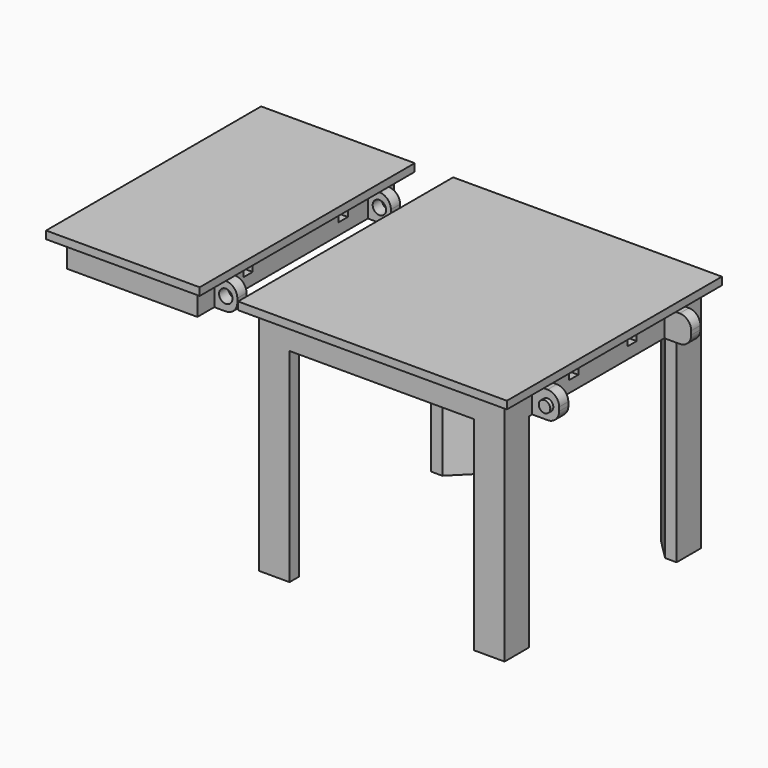
from build123d import *

# Parameters (mm, degrees)
F0_W      = 3
F0_H      = 50
F0_W_2    = 48
F0_H_2    = 3
F0_H_3    = 40
F1_DEPTH  = 2
F2_DEPTH  = 60
F0_W_3    = 4
F3_DEPTH  = 7
F4_R      = 1.25
F4_R_2    = 1.5
F5_DEPTH  = 1
F6_R      = 1.25
F6_R_2    = 1.5
F7_DEPTH  = 1
F8_W      = 28
F8_H      = 58
F8_W_2    = 3
F8_H_2    = 47
F8_H_3    = 3
F9_DEPTH  = 2
F10_DEPTH = 7
F11_DEPTH = 7
F12_R     = 1.75
F13_DEPTH = 61.501
F14_W     = 3
F14_H     = 4
F15_DEPTH = 52.7474034429
F16_R     = 3
F16_2_R   = 3
F17_R     = 2.99999
F17_2_R   = 2.99999
F18_W     = 3
F18_H     = 4
F19_DEPTH = 33.2525965571


# Not quite as in the source:
# - a fillet or chamfer is up to 0.001 mm smaller than in the source, because OpenCascade refuses the exact size


with BuildPart() as f1:
    # F0 (on Top) → F1 (new body)
    with BuildSketch(Plane.XY):
        Polygon((11, -6), (6, -11), (6, -59), (11, -64), (59, -64), (64, -59), (64, -11), (59, -6), align=None)
        with Locations((35.2474034429, -35)):
            Rectangle(F0_W, F0_H, mode=Mode.SUBTRACT)
        Polygon((67, -15), (67, -12), (67, -11), (64, -11), (64, -59), (67, -59), (67, -58), (67, -55), align=None)
        Polygon((70, 0), (0, 0), (0, -12), (3, -12), (3, -11), (3, -3), (11, -3), (59, -3), (67, -3), (67, -11), (67, -12), (70, -12), align=None)
        Polygon((3, -11), (3, -12), (3, -15), (3, -55), (3, -58), (3, -59), (6, -59), (6, -11), align=None)
        with Locations((35, -65.5)):
            Rectangle(F0_W_2, F0_H_2)
        Polygon((67, -59), (64, -59), (59, -64), (59, -67), (67, -67), align=None)
        Polygon((11, -64), (6, -59), (3, -59), (3, -67), (11, -67), align=None)
        Polygon((64, -11), (67, -11), (67, -3), (59, -3), (59, -6), align=None)
        with Locations((35, -4.5)):
            Rectangle(F0_W_2, F0_H_2)
        Polygon((3, -3), (3, -11), (6, -11), (11, -6), (11, -3), align=None)
        with Locations((68.5, -35)):
            Rectangle(F0_W, F0_H_3)
        with Locations((68.5, -13.5)):
            Rectangle(F0_W, F0_H_2)
        with Locations((68.5, -56.5)):
            Rectangle(F0_W, F0_H_2)
        Polygon((3, -58), (0, -58), (0, -70), (70, -70), (70, -58), (67, -58), (67, -59), (67, -67), (59, -67), (11, -67), (3, -67), (3, -59), align=None)
        with Locations((1.5, -35)):
            Rectangle(F0_W, F0_H_3)
        with Locations((1.5, -56.5)):
            Rectangle(F0_W, F0_H_2)
        with Locations((1.5, -13.5)):
            Rectangle(F0_W, F0_H_2)
        with Locations((35.2474034429, -35)):
            Rectangle(F0_W, F0_H)
    extrude(amount=F1_DEPTH)

    # F0 (on Top) → F2 (join)
    with BuildSketch(Plane.XY):
        Polygon((67, -59), (64, -59), (59, -64), (59, -67), (67, -67), align=None)
        Polygon((64, -11), (67, -11), (67, -3), (59, -3), (59, -6), align=None)
        Polygon((3, -3), (3, -11), (6, -11), (11, -6), (11, -3), align=None)
        Polygon((11, -64), (6, -59), (3, -59), (3, -67), (11, -67), align=None)
    extrude(amount=-F2_DEPTH)

    # F0 (on Top) → F3 (join)
    with BuildSketch(Plane.XY):
        Polygon((3, -11), (3, -12), (3, -15), (3, -55), (3, -58), (3, -59), (6, -59), (6, -11), align=None)
        with Locations((-2, -56.5)):
            Rectangle(F0_W_3, F0_H_2)
        with Locations((1.5, -56.5)):
            Rectangle(F0_W, F0_H_2)
        with Locations((1.5, -13.5)):
            Rectangle(F0_W, F0_H_2)
        with Locations((-2, -13.5)):
            Rectangle(F0_W_3, F0_H_2)
        with Locations((35, -65.5)):
            Rectangle(F0_W_2, F0_H_2)
        Polygon((67, -15), (67, -12), (67, -11), (64, -11), (64, -59), (67, -59), (67, -58), (67, -55), align=None)
        with Locations((68.5, -56.5)):
            Rectangle(F0_W, F0_H_2)
        with Locations((72, -56.5)):
            Rectangle(F0_W_3, F0_H_2)
        with Locations((72, -13.5)):
            Rectangle(F0_W_3, F0_H_2)
        with Locations((68.5, -13.5)):
            Rectangle(F0_W, F0_H_2)
        with Locations((35, -4.5)):
            Rectangle(F0_W_2, F0_H_2)
        with Locations((35.2474034429, -35)):
            Rectangle(F0_W, F0_H)
    extrude(amount=-F3_DEPTH)

    # F4 (on face) → F5 (join)
    with BuildSketch(Plane(origin=(0, -12, 0), x_dir=(-1, 0, 0), z_dir=(0, 1, 0))):
        with Locations((1, -3.5)):
            Circle(F4_R)
        with Locations((-71, -3.5)):
            Circle(F4_R_2)
    extrude(amount=F5_DEPTH)

    # F6 (on face) → F7 (join)
    with BuildSketch(Plane.XZ.offset(58)):
        with Locations((0, -3.5)):
            Circle(F6_R)
        with Locations((71, -3.5)):
            Circle(F6_R_2)
    extrude(amount=F7_DEPTH)


with BuildPart() as f9:
    # F8 (on Top) → F9 (new body)
    with BuildSketch(Plane.XY):
        Polygon((-13, -11.5), (-13, -8.5), (-13, -3), (-47, -3), (-47, -67), (-13, -67), (-13, -61.5), (-13, -58.5), align=None)
        with Locations((-30, -35)):
            Rectangle(F8_W, F8_H, mode=Mode.SUBTRACT)
        with Locations((-30, -35)):
            Rectangle(F8_W, F8_H)
        Polygon((-10, -8.5), (-10, 0), (-50, 0), (-50, -70), (-10, -70), (-10, -61.5), (-13, -61.5), (-13, -67), (-47, -67), (-47, -3), (-13, -3), (-13, -8.5), align=None)
        with Locations((-11.5, -35)):
            Rectangle(F8_W_2, F8_H_2)
        with Locations((-11.5, -60)):
            Rectangle(F8_W_2, F8_H_3)
        with Locations((-11.5, -10)):
            Rectangle(F8_W_2, F8_H_3)
    extrude(amount=F9_DEPTH)

    # F8 (on Top) → F10 (join)
    with BuildSketch(Plane.XY):
        Polygon((-13, -11.5), (-13, -8.5), (-13, -3), (-47, -3), (-47, -67), (-13, -67), (-13, -61.5), (-13, -58.5), align=None)
        with Locations((-30, -35)):
            Rectangle(F8_W, F8_H, mode=Mode.SUBTRACT)
    extrude(amount=-F10_DEPTH)

    # F8 (on Top) → F11 (join)
    with BuildSketch(Plane.XY):
        with Locations((-11.5, -60)):
            Rectangle(F8_W_2, F8_H_3)
        with Locations((-8.5, -60)):
            Rectangle(F8_W_2, F8_H_3)
        with Locations((-8.5, -10)):
            Rectangle(F8_W_2, F8_H_3)
        with Locations((-11.5, -10)):
            Rectangle(F8_W_2, F8_H_3)
    extrude(amount=-F11_DEPTH)

    # F12 (on face) → F13 (cut, through all)
    with BuildSketch(Plane.XZ.offset(61.5)):
        with Locations((-10, -3.5)):
            Circle(F12_R)
    extrude(amount=-F13_DEPTH, mode=Mode.SUBTRACT)


with BuildPart() as f15_tool:
    # F14 (on face) → F15 (new body, through all)
    with BuildSketch(Plane(origin=(-16, 0, 0), x_dir=(0, -1, 0), z_dir=(-1, 0, 0))):
        with Locations((50.5, -2)):
            Rectangle(F14_W, F14_H)
        with Locations((19.5, -2)):
            Rectangle(F14_W, F14_H)
    extrude(amount=-F15_DEPTH)


with BuildPart() as f1_1:
    add(f1.part)

    # F15: cut by f15_tool
    add(f15_tool.part, mode=Mode.SUBTRACT)

    # F16#2
    f16_2_edges = [f1_1.edges().sort_by_distance(p)[0] for p in [
        (-4, -13.5, -7),
        (-4, -56.5, -7),
        (74, -13.5, -7),
        (74, -56.5, -7),
    ]]
    fillet(f16_2_edges, radius=F16_2_R)

    # F17 (radius 3 in the source; OpenCascade refuses exactly that, so slightly less here)
    f17_edges = [f1_1.edges().sort_by_distance(p)[0] for p in [
        (-4, -13.5, 0),
        (-4, -56.5, 0),
        (74, -13.5, 0),
        (74, -56.5, 0),
    ]]
    fillet(f17_edges, radius=F17_R)

    # F18 (on face) → F19 (cut, through all)
    with BuildSketch(Plane.YZ.offset(67)):
        with Locations((-44.5, -2)):
            Rectangle(F18_W, F18_H)
        with Locations((-25.5, -2)):
            Rectangle(F18_W, F18_H)
    extrude(amount=-F19_DEPTH, mode=Mode.SUBTRACT)


with BuildPart() as f9_1:
    add(f9.part)

    # F15: cut by f15_tool
    add(f15_tool.part, mode=Mode.SUBTRACT)

    # F16
    f16_edges = [f9_1.edges().sort_by_distance(p)[0] for p in [
        (-7, -10, -7),
        (-7, -60, -7),
    ]]
    fillet(f16_edges, radius=F16_R)

    # F17#2 (radius 3 in the source; OpenCascade refuses exactly that, so slightly less here)
    f17_2_edges = [f9_1.edges().sort_by_distance(p)[0] for p in [
        (-7, -60, 0),
        (-7, -10, 0),
    ]]
    fillet(f17_2_edges, radius=F17_2_R)


solid = Compound([f1_1.part, f9_1.part])
